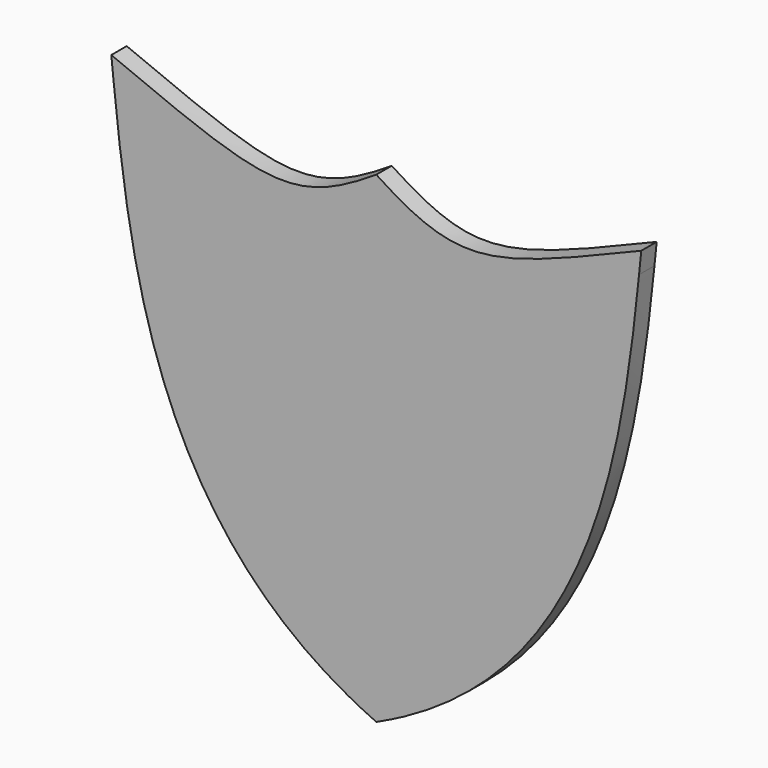
from build123d import *

# Parameters (mm, degrees)
F1_DEPTH = 5.08


# Not quite as in the source:
# - ends of sketch curves that miss each other by under 0.0002 mm in the source are joined


with BuildPart() as f1:
    # F0 (on Front) → F1 (new body)
    with BuildSketch(Plane.XZ):
        with BuildLine():
            add(Edge.make_bspline(
                [(69.85, 59.9050451917), (69.6591630317, 58.0205304518), (69.4657837415, 56.105507858), (69.2658161809, 54.1639224361)],
                knots=[0, 0, 0, 0, 6.3686924223, 6.3686924223, 6.3686924223, 6.3686924223], degree=3))
            add(Edge.make_bspline(
                [(69.85, 59.9050451917), (29.6646114439, 43.1978777051), (22.2865504252, 40.336203924), (0, 54.8465235897)],
                knots=[0, 0, 0, 0, 70.0329289749, 70.0329289749, 70.0329289749, 70.0329289749], degree=3))
            add(Edge.make_bspline(
                [(-69.85, 59.9050451917), (-29.6646114439, 43.1978777051), (-22.2865504252, 40.336203924), (0, 54.8465235897)],
                knots=[0, 0, 0, 0, 70.0329289749, 70.0329289749, 70.0329289749, 70.0329289749], degree=3))
            add(Edge.make_bspline(
                [(-69.85, 59.9050451917), (-69.6591630317, 58.0205304518), (-69.4657837415, 56.105507858), (-69.2658161809, 54.1639224361)],
                knots=[0, 0, 0, 0, 6.3686924223, 6.3686924223, 6.3686924223, 6.3686924223], degree=3))
            add(Edge.make_bspline(
                [(-69.2658161783, 54.1639224373), (-68.435377118, 53.8183422364), (-66.6556116111, 53.0753974425), (-64.8761610511, 52.3317704272), (-63.9263795957, 51.9355805251)],
                knots=[2.7434490873, 2.7434490873, 2.7434490873, 2.7434490873, 5.4418546999, 8.5291588217, 8.5291588217, 8.5291588217, 8.5291588217], degree=3))
            add(Edge.make_bspline(
                [(-63.9263795957, 51.9355805251), (-61.8621309574, 51.0745040519), (-56.1021142689, 48.6812764055), (-47.7406374178, 45.3549636264), (-39.4375160633, 42.5935516843), (-33.4464354817, 41.219419811), (-28.7724481834, 40.4865030944), (-24.7049900131, 40.2576737616), (-20.7256507732, 40.4650803867), (-16.8202071601, 41.130682749), (-12.9707995749, 42.2328724248), (-8.7178720085, 43.9515281326), (-4.3615220824, 46.044445106), (-1.3844475727, 47.8958436146), (-0.0332400038, 48.7623797008), (0, 48.7837122639)],
                knots=[8.5291588217, 8.5291588217, 8.5291588217, 8.5291588217, 15.2390848713, 27.2415659858, 35.5219361762, 41.4579165876, 45.6606303606, 49.7014880209, 53.6563538897, 57.5892253523, 61.5614465465, 65.6429176226, 71.3392641934, 76.0338793574, 76.152307097, 76.152307097, 76.152307097, 76.152307097], degree=3))
            add(Edge.make_bspline(
                [(63.9263795957, 51.9355805251), (61.8621309574, 51.0745040519), (56.1021142689, 48.6812764055), (47.7406374178, 45.3549636264), (39.4375160633, 42.5935516843), (33.4464354817, 41.219419811), (28.7724481834, 40.4865030944), (24.7049900131, 40.2576737616), (20.7256507732, 40.4650803867), (16.8202071601, 41.130682749), (12.9707995749, 42.2328724248), (8.7178720085, 43.9515281326), (4.3615220824, 46.044445106), (1.3844475727, 47.8958436146), (0.0332400038, 48.7623797008), (0, 48.7837122639)],
                knots=[8.5291588217, 8.5291588217, 8.5291588217, 8.5291588217, 15.2390848713, 27.2415659858, 35.5219361762, 41.4579165876, 45.6606303606, 49.7014880209, 53.6563538897, 57.5892253523, 61.5614465465, 65.6429176226, 71.3392641934, 76.0338793574, 76.152307097, 76.152307097, 76.152307097, 76.152307097], degree=3))
            add(Edge.make_bspline(
                [(69.2658161783, 54.1639224373), (68.435377118, 53.8183422364), (66.6556116111, 53.0753974425), (64.8761610511, 52.3317704272), (63.9263795957, 51.9355805251)],
                knots=[2.7434490873, 2.7434490873, 2.7434490873, 2.7434490873, 5.4418546999, 8.5291588217, 8.5291588217, 8.5291588217, 8.5291588217], degree=3))
        make_face()
        with BuildLine():
            add(Edge.make_bspline(
                [(69.2658161809, 54.1639224361), (64.7750418343, 10.5607401093), (56.961539529, -46.4391375943), (0, -72.1534764103)],
                knots=[6.3686924223, 6.3686924223, 6.3686924223, 6.3686924223, 149.3936934001, 149.3936934001, 149.3936934001, 149.3936934001], degree=3))
            add(Edge.make_bspline(
                [(69.2658161809, 54.1639224361), (68.435377118, 53.8183422364), (66.6556116111, 53.0753974425), (64.8761610511, 52.3317704272), (63.9263795957, 51.9355805251)],
                knots=[2.7434490873, 2.7434490873, 2.7434490873, 2.7434490873, 5.4418546999, 8.5291588217, 8.5291588217, 8.5291588217, 8.5291588217], degree=3))
            add(Edge.make_bspline(
                [(63.9263795957, 51.9355805251), (63.6253355549, 49.0777517049), (62.6683683388, 40.3495230581), (60.6243910667, 25.2903357755), (56.8644266428, 6.9882226507), (51.2318594545, -10.9343345603), (43.1811515415, -27.8959051236), (32.1695249216, -43.368046578), (18.0779778329, -56.4464882841), (6.2692486092, -63.5700966147), (1.35086e-05, -66.5543592491)],
                knots=[0.0627067414, 0.0627067414, 0.0627067414, 0.0627067414, 0.125, 0.25, 0.375, 0.5, 0.625, 0.75, 0.875, 0.9876294304, 0.9876294304, 0.9876294304, 0.9876294304], degree=3))
            add(Edge.make_bspline(
                [(-63.9263795983, 51.9355805238), (-63.6253355549, 49.0777517049), (-62.6683683388, 40.3495230581), (-60.6243910667, 25.2903357755), (-56.8644266428, 6.9882226507), (-51.2318594545, -10.9343345603), (-43.1811515415, -27.8959051236), (-32.1695249216, -43.368046578), (-18.0779778329, -56.4464882841), (-6.2692486092, -63.5700966147), (1.35086e-05, -66.5543592491)],
                knots=[0.0627067414, 0.0627067414, 0.0627067414, 0.0627067414, 0.125, 0.25, 0.375, 0.5, 0.625, 0.75, 0.875, 0.9876294304, 0.9876294304, 0.9876294304, 0.9876294304], degree=3))
            add(Edge.make_bspline(
                [(-69.2658161783, 54.1639224373), (-68.435377118, 53.8183422364), (-66.6556116111, 53.0753974425), (-64.8761610511, 52.3317704272), (-63.9263795983, 51.9355805238)],
                knots=[2.7434490873, 2.7434490873, 2.7434490873, 2.7434490873, 5.4418546999, 8.5291588217, 8.5291588217, 8.5291588217, 8.5291588217], degree=3))
            add(Edge.make_bspline(
                [(-69.2658161783, 54.1639224373), (-64.7750418343, 10.5607401093), (-56.961539529, -46.4391375943), (0, -72.1534764103)],
                knots=[6.3686924223, 6.3686924223, 6.3686924223, 6.3686924223, 149.3936934001, 149.3936934001, 149.3936934001, 149.3936934001], degree=3))
        make_face()
        with BuildLine():
            add(Edge.make_bspline(
                [(63.9263795983, 51.9355805238), (63.6253355549, 49.0777517049), (62.6683683388, 40.3495230581), (60.6243910667, 25.2903357755), (56.8644266428, 6.9882226507), (51.2318594545, -10.9343345603), (43.1811515415, -27.8959051236), (32.1695249216, -43.368046578), (18.0779778329, -56.4464882841), (6.2692486092, -63.5700966147), (1.35086e-05, -66.5543592491)],
                knots=[0.0627067414, 0.0627067414, 0.0627067414, 0.0627067414, 0.125, 0.25, 0.375, 0.5, 0.625, 0.75, 0.875, 0.9876294304, 0.9876294304, 0.9876294304, 0.9876294304], degree=3))
            add(Edge.make_bspline(
                [(63.9263795983, 51.9355805238), (61.8621309574, 51.0745040519), (56.1021142689, 48.6812764055), (47.7406374178, 45.3549636264), (39.4375160633, 42.5935516843), (33.4464354817, 41.219419811), (28.7724481834, 40.4865030944), (24.7049900131, 40.2576737616), (20.7256507732, 40.4650803867), (16.8202071601, 41.130682749), (12.9707995749, 42.2328724248), (8.7178720085, 43.9515281326), (4.3615220824, 46.044445106), (1.3844475727, 47.8958436146), (0.0332400038, 48.7623797008), (0, 48.7837122639)],
                knots=[8.5291588217, 8.5291588217, 8.5291588217, 8.5291588217, 15.2390848713, 27.2415659858, 35.5219361762, 41.4579165876, 45.6606303606, 49.7014880209, 53.6563538897, 57.5892253523, 61.5614465465, 65.6429176226, 71.3392641934, 76.0338793574, 76.152307097, 76.152307097, 76.152307097, 76.152307097], degree=3))
            add(Edge.make_bspline(
                [(-63.9263795957, 51.9355805251), (-61.8621309574, 51.0745040519), (-56.1021142689, 48.6812764055), (-47.7406374178, 45.3549636264), (-39.4375160633, 42.5935516843), (-33.4464354817, 41.219419811), (-28.7724481834, 40.4865030944), (-24.7049900131, 40.2576737616), (-20.7256507732, 40.4650803867), (-16.8202071601, 41.130682749), (-12.9707995749, 42.2328724248), (-8.7178720085, 43.9515281326), (-4.3615220824, 46.044445106), (-1.3844475727, 47.8958436146), (-0.0332400038, 48.7623797008), (0, 48.7837122639)],
                knots=[8.5291588217, 8.5291588217, 8.5291588217, 8.5291588217, 15.2390848713, 27.2415659858, 35.5219361762, 41.4579165876, 45.6606303606, 49.7014880209, 53.6563538897, 57.5892253523, 61.5614465465, 65.6429176226, 71.3392641934, 76.0338793574, 76.152307097, 76.152307097, 76.152307097, 76.152307097], degree=3))
            add(Edge.make_bspline(
                [(-63.9263795957, 51.9355805251), (-63.6253355549, 49.0777517049), (-62.6683683388, 40.3495230581), (-60.6243910667, 25.2903357755), (-56.8644266428, 6.9882226507), (-51.2318594545, -10.9343345603), (-43.1811515415, -27.8959051236), (-32.1695249216, -43.368046578), (-18.0779778329, -56.4464882841), (-6.2692486092, -63.5700966147), (1.35086e-05, -66.5543592491)],
                knots=[0.0627067414, 0.0627067414, 0.0627067414, 0.0627067414, 0.125, 0.25, 0.375, 0.5, 0.625, 0.75, 0.875, 0.9876294304, 0.9876294304, 0.9876294304, 0.9876294304], degree=3))
        make_face()
    extrude(amount=F1_DEPTH)


solid = f1.part
